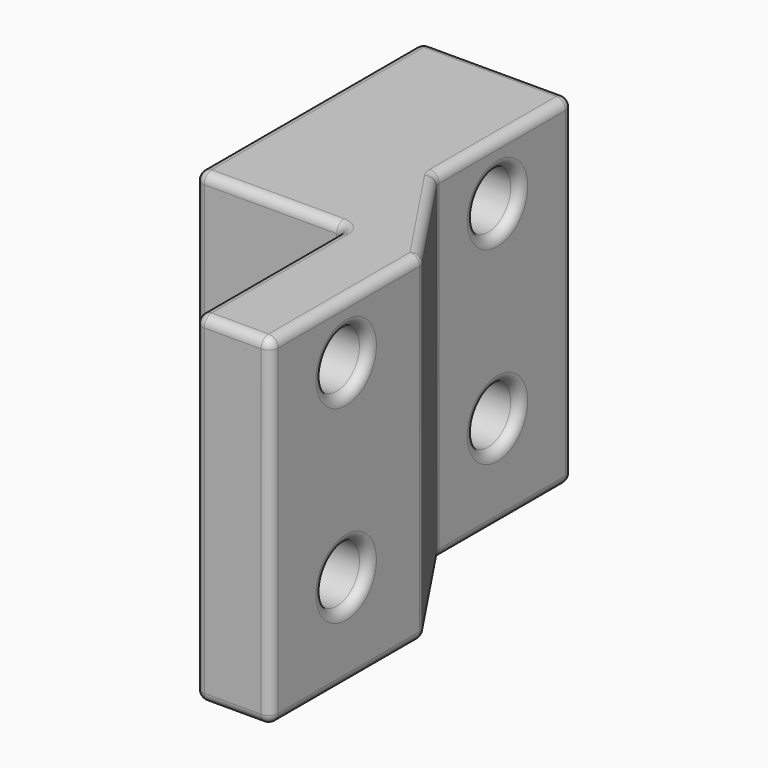
from build123d import *

# Parameters (mm, degrees)
F0_W     = 4
F0_H     = 10
F1_DEPTH = 18
F2_R     = 1.5
F3_DEPTH = 10
F4_DEPTH = 10
F5_F1_R  = 0.5
F5_F2_R  = 0.5


with BuildPart() as f1:
    # F0 (on Top) → F1 (new body)
    with BuildSketch(Plane.XY):
        Polygon((-4, 15), (-12, 15), (-12, 0), (-4, 0), (-4, 6), align=None)
        Polygon((0, 0), (-4, 6), (-4, 0), align=None)
        with Locations((-2, -5)):
            Rectangle(F0_W, F0_H)
    extrude(amount=F1_DEPTH)

    # F2 (on face) → F3 (cut, symmetric)
    with BuildSketch(Plane(origin=(-4, 0, 0), x_dir=(0, -1, 0), z_dir=(-1, 0, 0))):
        with Locations((5, 5)):
            Circle(F2_R)
        with Locations((5, 15)):
            Circle(F2_R)
    extrude(amount=F3_DEPTH, both=True, mode=Mode.SUBTRACT)

    # F2 (on face) → F4 (cut, symmetric)
    with BuildSketch(Plane(origin=(-4, 0, 0), x_dir=(0, -1, 0), z_dir=(-1, 0, 0))):
        with Locations((-10, 15)):
            Circle(F2_R)
        with Locations((-10, 5)):
            Circle(F2_R)
    extrude(amount=F4_DEPTH, both=True, mode=Mode.SUBTRACT)

    # F5: fillet of radius 0.5 on 28 edges, made by hand

    # F5_f1
    f5_f1_edges = [f1.edges().sort_by_distance(p)[0] for p in [
        (-4, 6, 9),
        (-4, 0, 9),
    ]]
    fillet(f5_f1_edges, radius=F5_F1_R)

    # F5_f2
    f5_f2_edges = [f1.edges().sort_by_distance(p)[0] for p in [
        (-4, 10.5756939094, 0),
        (-4, 10.5756939094, 18),
        (-4, 15, 9),
        (-4, 11.5, 15),
        (-4, 11.5, 5),
        (0, -10, 9),
        (0, -5, 0),
        (0, -5, 18),
        (0, 0, 9),
        (0, -3.5, 15),
        (0, -3.5, 5),
        (-4, -10, 9),
        (-2, -10, 0),
        (-2, -10, 18),
        (-4, -5.25, 0),
        (-4, -5.25, 18),
        (-4, -3.5, 15),
        (-4, -3.5, 5),
        (-12, 15, 9),
        (-12, 7.5, 0),
        (-12, 7.5, 18),
        (-12, 0, 9),
        (-12, 11.5, 15),
        (-12, 11.5, 5),
        (-8, 15, 0),
        (-8, 15, 18),
        (-4.1464466094, -0.1464466094, 18),
        (-4.1464466094, -0.1464466094, 0),
        (-3.9785460132, 6.0064957445, 18),
        (-3.9785460132, 6.0064957445, 0),
    ]]
    fillet(f5_f2_edges, radius=F5_F2_R)


solid = f1.part
